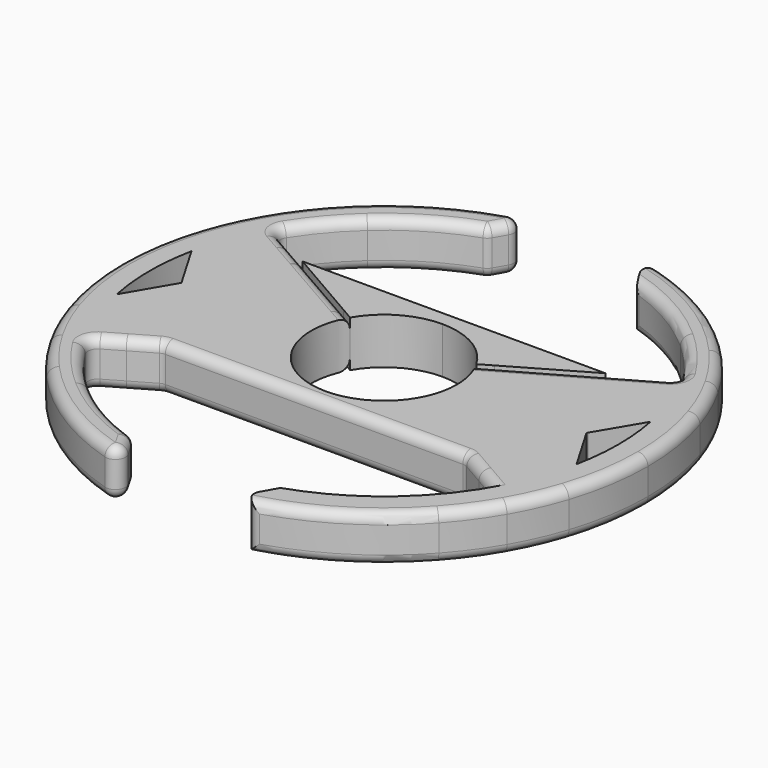
from build123d import *

# Parameters (mm, degrees)
F1_DEPTH = 7
F2_F1_R  = 1.5
F2_F2_R  = 1.5


with BuildPart() as f1:
    # F0 (on Top) → F1 (new body)
    with BuildSketch(Plane.XY):
        with BuildLine():
            Line((-11.4884131462, -6.6328384225), (-9.5262794416, -5.5))
            ThreePointArc((-9.5262794416, -5.5), (-10.9999880296, -0.0162280005), (-9.5424659579, 5.4718683685))
            Line((-9.5424659579, 5.4718683685), (-11.4494710487, 6.5653887311))
            Line((-11.4494710487, 6.5653887311), (-15.2660056991, -0.0450431922))
            Line((-15.2660056991, -0.0450431922), (-11.4884131462, -6.6328384225))
        make_face()
        with BuildLine():
            ThreePointArc((9.5583523485, 5.4440702036), (10.6334819282, 2.8158590311), (11, 0))
            ThreePointArc((11, 0), (10.6251840892, -2.8470094961), (9.5262794416, -5.5))
            Line((9.5262794416, -5.5), (11.4884131462, -6.6328384225))
            Line((11.4884131462, -6.6328384225), (15.2660056991, -0.0450431922))
            Line((15.2660056991, -0.0450431922), (11.4686793157, 6.5321190369))
            Line((11.4686793157, 6.5321190369), (9.5583523485, 5.4440702036))
        make_face()
        with BuildLine():
            Line((0, -13.1982271537), (0, -11))
            ThreePointArc((0, -11), (-5.5, -9.5262794416), (-9.5262794416, -5.5))
            Line((-9.5262794416, -5.5), (-11.4884131462, -6.6328384225))
            Line((-11.4884131462, -6.6328384225), (-7.7236689927, -13.1982271537))
            Line((-7.7236689927, -13.1982271537), (0, -13.1982271537))
        make_face()
        with BuildLine():
            Line((11.4884131462, -6.6328384225), (9.5262794416, -5.5))
            ThreePointArc((9.5262794416, -5.5), (5.5, -9.5262794416), (0, -11))
            Line((0, -11), (0, -13.1982271537))
            Line((0, -13.1982271537), (7.7236689927, -13.1982271537))
            Line((7.7236689927, -13.1982271537), (11.4884131462, -6.6328384225))
        make_face()
        Polygon((-15.2660056991, -0.0450431922), (-11.4494710487, 6.5653887311), (-22.783297147, 13.064464001), align=None)
        Polygon((-22.86, -13.1982271537), (-11.4884131462, -6.6328384225), (-15.2660056991, -0.0450431922), align=None)
        with BuildLine():
            ThreePointArc((-22.8988424216, 13.1307203059), (-26.3964255823, -0.0389419703), (-22.86, -13.1982271537))
            Line((-22.86, -13.1982271537), (-15.2660056991, -0.0450431922))
            Line((-15.2660056991, -0.0450431922), (-22.783297147, 13.064464001))
            Line((-22.783297147, 13.064464001), (-22.8988424216, 13.1307203059))
        make_face()
        with BuildLine():
            Line((22.7083848356, 12.9338233984), (15.2660056991, -0.0450431922))
            Line((15.2660056991, -0.0450431922), (22.86, -13.1982271537))
            ThreePointArc((22.86, -13.1982271537), (25.4970169379, -6.8319050979), (26.3964543073, 0))
            ThreePointArc((26.3964543073, 0), (25.5169290768, 6.7571540228), (22.9369646383, 13.0640136705))
            Line((22.9369646383, 13.0640136705), (22.7083848356, 12.9338233984))
        make_face()
        Polygon((22.7083848356, 12.9338233984), (11.4686793157, 6.5321190369), (15.2660056991, -0.0450431922), align=None)
        Polygon((15.2660056991, -0.0450431922), (11.4884131462, -6.6328384225), (22.86, -13.1982271537), align=None)
        Polygon((-7.7236689927, -13.1982271537), (-11.4884131462, -6.6328384225), (-22.86, -13.1982271537), align=None)
        Polygon((22.86, -13.1982271537), (11.4884131462, -6.6328384225), (7.7236689927, -13.1982271537), align=None)
        with BuildLine():
            Line((-30.7342490519, 0.2560747826), (-30.5840239918, -0.0006066234))
            Line((-30.5840239918, -0.0006066234), (-22.8993387832, 13.131004931))
            Line((-22.8993387832, 13.131004931), (-26.6627913636, 15.2890547707))
            ThreePointArc((-26.6627913636, 15.2890547707), (-29.6665246355, 8.0347342915), (-30.7342490519, 0.2560747826))
        make_face()
        with BuildLine():
            Line((-26.6175643009, -15.3676579143), (-22.86, -13.1982271537))
            Line((-22.86, -13.1982271537), (-30.5840239918, -0.0006066234))
            Line((-30.5840239918, -0.0006066234), (-30.7342388675, -0.2572942227))
            ThreePointArc((-30.7342388675, -0.2572942227), (-29.6544786565, -8.0790800647), (-26.6175643009, -15.3676579143))
        make_face()
        with BuildLine():
            Line((-30.5840239918, -0.0006066234), (-22.86, -13.1982271537))
            ThreePointArc((-22.86, -13.1982271537), (-26.3964255823, -0.0389419703), (-22.8988424216, 13.1307203059))
            Line((-22.8988424216, 13.1307203059), (-22.8993387832, 13.131004931))
            Line((-22.8993387832, 13.131004931), (-30.5840239918, -0.0006066234))
        make_face()
        with BuildLine():
            Line((22.9381479847, 13.0646876591), (30.6356845324, -0.0888842995))
            Line((30.6356845324, -0.0888842995), (30.7352145126, 0.0789173429))
            ThreePointArc((30.7352145126, 0.0789173429), (29.7010950851, 7.9059844312), (26.7071798393, 15.2113833727))
            Line((26.7071798393, 15.2113833727), (22.9381479847, 13.0646876591))
        make_face()
        with BuildLine():
            ThreePointArc((26.3964543073, 0), (25.4970169379, -6.8319050979), (22.86, -13.1982271537))
            Line((22.86, -13.1982271537), (30.6356845324, -0.0888842995))
            Line((30.6356845324, -0.0888842995), (22.9381479847, 13.0646876591))
            Line((22.9381479847, 13.0646876591), (22.9369646383, 13.0640136705))
            ThreePointArc((22.9369646383, 13.0640136705), (25.5169290768, 6.7571540228), (26.3964543073, 0))
        make_face()
        with BuildLine():
            Line((30.6356845324, -0.0888842995), (22.86, -13.1982271537))
            Line((22.86, -13.1982271537), (26.6175643009, -15.3676579143))
            ThreePointArc((26.6175643009, -15.3676579143), (29.6544786565, -8.0790800647), (30.7342388675, -0.2572942227))
            Line((30.7342388675, -0.2572942227), (30.6356845324, -0.0888842995))
        make_face()
        with BuildLine():
            ThreePointArc((26.7071798393, 15.2113833727), (29.7010950851, 7.9059844312), (30.7352145126, 0.0789173429))
            Line((30.7352145126, 0.0789173429), (34.7550959877, 6.8561990434))
            ThreePointArc((34.7550959877, 6.8561990434), (33.2005715794, 12.355007456), (30.7821600075, 17.5323354893))
            Line((30.7821600075, 17.5323354893), (26.7071798393, 15.2113833727))
        make_face()
        with BuildLine():
            ThreePointArc((30.7821600075, 17.5323354893), (33.2005715794, 12.355007456), (34.7550959877, 6.8561990434))
            Line((34.7550959877, 6.8561990434), (37.9275745015, 12.2048096207))
            ThreePointArc((37.9275745015, 12.2048096207), (36.4684072184, 16.0472290568), (34.6211517556, 19.71887767))
            Line((34.6211517556, 19.71887767), (30.7821600075, 17.5323354893))
        make_face()
        with BuildLine():
            ThreePointArc((34.7145143201, -7.0588000364), (33.1277647383, -12.5489189128), (30.6788709347, -17.7124543926))
            Line((30.6788709347, -17.7124543926), (34.504981004, -19.921460071))
            ThreePointArc((34.504981004, -19.921460071), (36.3738579229, -16.2604042155), (37.855591549, -12.4262815808))
            Line((37.855591549, -12.4262815808), (34.7145143201, -7.0588000364))
        make_face()
        with BuildLine():
            ThreePointArc((30.7342388675, -0.2572942227), (29.6544786565, -8.0790800647), (26.6175643009, -15.3676579143))
            Line((26.6175643009, -15.3676579143), (30.6788709347, -17.7124543926))
            ThreePointArc((30.6788709347, -17.7124543926), (33.1277647383, -12.5489189128), (34.7145143201, -7.0588000364))
            Line((34.7145143201, -7.0588000364), (30.7342388675, -0.2572942227))
        make_face()
        with BuildLine():
            Line((-30.6788709347, -17.7124543926), (-26.6175643009, -15.3676579143))
            ThreePointArc((-26.6175643009, -15.3676579143), (-29.6544786565, -8.0790800647), (-30.7342388675, -0.2572942227))
            Line((-30.7342388675, -0.2572942227), (-34.7145143201, -7.0588000364))
            ThreePointArc((-34.7145143201, -7.0588000364), (-33.1277647383, -12.5489189128), (-30.6788709347, -17.7124543926))
        make_face()
        with BuildLine():
            Line((-34.504981004, -19.921460071), (-30.6788709347, -17.7124543926))
            ThreePointArc((-30.6788709347, -17.7124543926), (-33.1277647383, -12.5489189128), (-34.7145143201, -7.0588000364))
            Line((-34.7145143201, -7.0588000364), (-37.855591549, -12.4262815808))
            ThreePointArc((-37.855591549, -12.4262815808), (-36.3738579229, -16.2604042155), (-34.504981004, -19.921460071))
        make_face()
        with BuildLine():
            Line((-37.8560868788, 12.4247724999), (-34.7147952958, 7.0574180833))
            ThreePointArc((-34.7147952958, 7.0574180833), (-33.1464905664, 12.4993730069), (-30.7309987404, 17.6218579852))
            Line((-30.7309987404, 17.6218579852), (-34.56360992, 19.8195649485))
            ThreePointArc((-34.56360992, 19.8195649485), (-36.3981298963, 16.2059996761), (-37.8560868788, 12.4247724999))
        make_face()
        with BuildLine():
            Line((-34.7147952958, 7.0574180833), (-30.7342490519, 0.2560747826))
            ThreePointArc((-30.7342490519, 0.2560747826), (-29.6665246355, 8.0347342915), (-26.6627913636, 15.2890547707))
            Line((-26.6627913636, 15.2890547707), (-30.7309987404, 17.6218579852))
            ThreePointArc((-30.7309987404, 17.6218579852), (-33.1464905664, 12.4993730069), (-34.7147952958, 7.0574180833))
        make_face()
        with BuildLine():
            ThreePointArc((-30.7309987404, 17.6218579852), (-27.5299511629, 22.2940788418), (-23.6252272462, 26.3964543073))
            Line((-23.6252272462, 26.3964543073), (-29.8443543312, 26.3964543073))
            ThreePointArc((-29.8443543312, 26.3964543073), (-32.3714431738, 23.2281715228), (-34.56360992, 19.8195649485))
            Line((-34.56360992, 19.8195649485), (-30.7309987404, 17.6218579852))
        make_face()
        with BuildLine():
            Line((34.504981004, -19.921460071), (30.6788709347, -17.7124543926))
            ThreePointArc((30.6788709347, -17.7124543926), (27.3675522542, -22.4931377546), (23.3186876658, -26.6676389652))
            Line((23.3186876658, -26.6676389652), (29.6022856799, -26.6676389652))
            ThreePointArc((29.6022856799, -26.6676389652), (32.2306243011, -23.4231753315), (34.504981004, -19.921460071))
        make_face()
        with BuildLine():
            ThreePointArc((-23.3186876658, -26.6676389652), (-27.3675522542, -22.4931377546), (-30.6788709347, -17.7124543926))
            Line((-30.6788709347, -17.7124543926), (-34.504981004, -19.921460071))
            ThreePointArc((-34.504981004, -19.921460071), (-32.2306243011, -23.4231753315), (-29.6022856799, -26.6676389652))
            Line((-29.6022856799, -26.6676389652), (-23.3186876658, -26.6676389652))
        make_face()
        with BuildLine():
            ThreePointArc((23.6252272462, 26.3964543073), (27.5623674155, 22.2539898644), (30.7821600075, 17.5323354893))
            Line((30.7821600075, 17.5323354893), (34.6211517556, 19.71887767))
            ThreePointArc((34.6211517556, 19.71887767), (32.4052137193, 23.1810355518), (29.8443543312, 26.3964543074))
            Line((29.8443543312, 26.3964543073), (23.6252272462, 26.3964543073))
        make_face()
        with BuildLine():
            ThreePointArc((35.4249087851, 0), (35.246862738, -3.5472284339), (34.7145143201, -7.0588000364))
            Line((34.7145143201, -7.0588000364), (37.855591549, -12.4262815808))
            ThreePointArc((37.855591549, -12.4262815808), (39.3429510616, -6.2920972033), (39.8429201421, 0))
            ThreePointArc((39.8429201421, 0), (39.36117127, 6.1770933051), (37.9275745015, 12.2048096207))
            Line((37.9275745015, 12.2048096207), (34.7550959877, 6.8561990434))
            ThreePointArc((34.7550959877, 6.8561990434), (35.257057929, 3.444419926), (35.4249087851, 0))
        make_face()
        with BuildLine():
            Line((-37.855591549, -12.4262815808), (-34.7145143201, -7.0588000364))
            ThreePointArc((-34.7145143201, -7.0588000364), (-35.4249087781, -0.0007051138), (-34.7147952958, 7.0574180833))
            Line((-34.7147952958, 7.0574180833), (-37.8560868788, 12.4247724999))
            ThreePointArc((-37.8560868788, 12.4247724999), (-39.8429201342, -0.0007941468), (-37.855591549, -12.4262815808))
        make_face()
        with BuildLine():
            ThreePointArc((-11.2441570083, -33.5930512994), (-17.6249224677, -30.729241293), (-23.3186876658, -26.6676389652))
            Line((-23.3186876658, -26.6676389652), (-29.6022856799, -26.6676389652))
            ThreePointArc((-29.6022856799, -26.6676389652), (-19.8650562602, -34.53748435), (-8.1663202509, -38.9970447471))
            Line((-8.1663202509, -38.9970447471), (-11.2441570083, -33.5930512994))
        make_face()
        with BuildLine():
            Line((29.6022856799, -26.6676389652), (23.3186876658, -26.6676389652))
            ThreePointArc((23.3186876658, -26.6676389652), (17.6249224677, -30.729241293), (11.2441570083, -33.5930512994))
            Line((11.2441570083, -33.5930512994), (8.1663202509, -38.9970447471))
            ThreePointArc((8.1663202509, -38.9970447471), (19.8650562602, -34.53748435), (29.6022856799, -26.6676389652))
        make_face()
        with BuildLine():
            ThreePointArc((11.2441570083, 33.5930512994), (17.8021414902, 30.6269149735), (23.6252272462, 26.3964543073))
            Line((23.6252272462, 26.3964543073), (29.8443543312, 26.3964543073))
            ThreePointArc((29.8443543312, 26.3964543074), (20.0224015893, 34.4465051935), (8.1663202509, 38.9970447471))
            Line((8.1663202509, 38.9970447471), (11.2441570083, 33.5930512994))
        make_face()
        with BuildLine():
            ThreePointArc((-23.6252272462, 26.3964543073), (-17.8021414902, 30.6269149735), (-11.2441570083, 33.5930512994))
            Line((-11.2441570083, 33.5930512994), (-8.1663202509, 38.9970447471))
            ThreePointArc((-8.1663202509, 38.9970447471), (-20.0224015893, 34.4465051935), (-29.8443543312, 26.3964543073))
            Line((-29.8443543312, 26.3964543073), (-23.6252272462, 26.3964543073))
        make_face()
    extrude(amount=F1_DEPTH)

    # F2: fillet of radius 1.5 on 28 edges, made by hand

    # F2_f1
    f2_f1_edges = [f1.edges().sort_by_distance(p)[0] for p in [
        (-22.86, -13.1982271537, 3.5),
        (22.86, -13.1982271537, 3.5),
        (-30.7309987404, 17.6218579852, 3.5),
        (-30.6788709347, -17.7124543926, 3.5),
        (30.7821600075, 17.5323354893, 3.5),
    ]]
    fillet(f2_f1_edges, radius=F2_F1_R)

    # F2_f2
    f2_f2_edges = [f1.edges().sort_by_distance(p)[0] for p in [
        (8.1663202509, -38.9970447471, 3.5),
        (8.1663202509, 38.9970447471, 3.5),
        (39.8429201421, 0, 0),
        (39.8429201421, 0, 7),
        (-8.1663202509, 38.9970447471, 3.5),
        (-8.1663202509, -38.9970447471, 3.5),
        (-39.8429201421, 0, 0),
        (-39.8429201421, 0, 7),
        (0, -13.1982271537, 0),
        (0, -13.1982271537, 7),
        (-11.2441570083, 33.5930512994, 3.5),
        (-21.8441162799, 27.888326346, 0),
        (-21.8441162799, 27.888326346, 7),
        (21.8846800716, 27.8565062525, 0),
        (-11.2441570083, -33.5930512994, 3.5),
        (-21.8029496203, -27.9205220275, 0),
        (-21.8029496203, -27.9205220275, 7),
        (-9.7052386296, -36.2950480233, 0),
        (-9.7052386296, -36.2950480233, 7),
        (-9.7052386296, 36.2950480233, 0),
        (-9.7052386296, 36.2950480233, 7),
        (11.2441570083, 33.5930512994, 3.5),
        (21.8846800716, 27.8565062525, 7),
        (30.1625528556, 17.7123251946, 7),
        (-30.0582194721, -17.8888093717, 7),
        (-30.0582194721, -17.8888093717, 0),
        (30.1625528556, 17.7123251946, 0),
        (-30.1108703222, 17.8000434551, 7),
        (-30.1108703222, 17.8000434551, 0),
        (-22.846304779, -13.2493384142, 7),
        (22.846304779, -13.2493384142, 7),
        (-22.846304779, -13.2493384142, 0),
        (22.846304779, -13.2493384142, 0),
    ]]
    fillet(f2_f2_edges, radius=F2_F2_R)


with BuildPart() as f1b:
    # F0 (on Top) → F1, piece 2 (new body)
    with BuildSketch(Plane.XY):
        with BuildLine():
            ThreePointArc((0, 11), (5.5, 9.5262794416), (9.5262794416, 5.5))
            Line((9.5262794416, 5.5), (11.43, 6.5991135768))
            Line((11.43, 6.5991135768), (7.62, 13.1982271537))
            Line((7.62, 13.1982271537), (0, 13.1982271537))
            Line((0, 13.1982271537), (0, 11))
        make_face()
        with BuildLine():
            ThreePointArc((-9.5262794416, 5.5), (-5.5, 9.5262794416), (0, 11))
            Line((0, 11), (0, 13.1982271537))
            Line((0, 13.1982271537), (-7.62, 13.1982271537))
            Line((-7.62, 13.1982271537), (-11.43, 6.5991135768))
            Line((-11.43, 6.5991135768), (-9.5262794416, 5.5))
        make_face()
        Polygon((-22.86, 13.1982271537), (-11.43, 6.5991135768), (-7.62, 13.1982271537), align=None)
        Polygon((7.62, 13.1982271537), (11.43, 6.5991135768), (22.86, 13.1982271537), align=None)
    extrude(amount=F1_DEPTH)


solid = Compound([f1.part, f1b.part])
